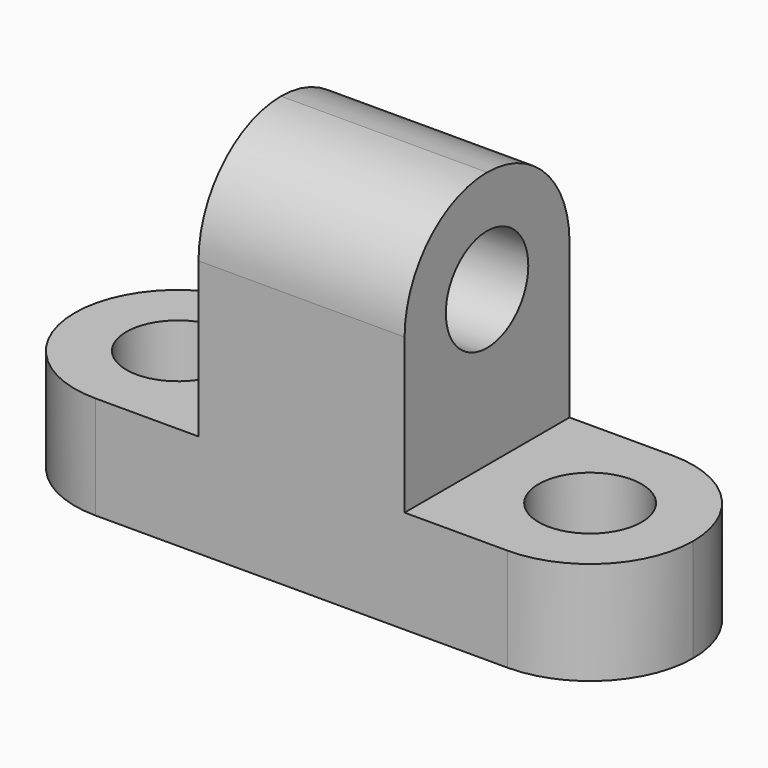
from build123d import *

# Parameters (mm, degrees)
F0_W      = 25.4
F0_H      = 44.45
F1_DEPTH  = 25.4
F2_R      = 12.69999
F3_W      = 25.4
F3_H      = 12.7
F4_DEPTH  = 25.4
F5_R      = 12.69999
F7_W      = 25.4
F7_H      = 12.7
F8_DEPTH  = 25.4
F9_R      = 12.69999
F11_R     = 6.35
F12_DEPTH = 25.4
F6_R      = 6.35
F13_DEPTH = 25.4
F10_R     = 6.35
F14_DEPTH = 25.4


# Not quite as in the source:
# - a fillet or chamfer is up to 0.001 mm smaller than in the source, because OpenCascade refuses the exact size


with BuildPart() as f1:
    # F0 (on Front) → F1 (new body)
    with BuildSketch(Plane.XZ):
        with Locations((12.7, 22.225)):
            Rectangle(F0_W, F0_H)
    extrude(amount=-F1_DEPTH)

    # F2 (radius 12.7 in the source; OpenCascade refuses exactly that, so slightly less here)
    f2_edges = [f1.edges().sort_by_distance(p)[0] for p in [
        (12.7, 0, 44.45),
        (12.7, 25.4, 44.45),
    ]]
    fillet(f2_edges, radius=F2_R)

    # F3 (on face) → F4 (join)
    with BuildSketch(Plane.YZ.offset(25.4)):
        with Locations((12.7, 6.35)):
            Rectangle(F3_W, F3_H)
    extrude(amount=F4_DEPTH)

    # F5 (radius 12.7 in the source; OpenCascade refuses exactly that, so slightly less here)
    f5_edges = [f1.edges().sort_by_distance(p)[0] for p in [
        (50.8, 0, 6.35),
        (50.8, 25.4, 6.35),
    ]]
    fillet(f5_edges, radius=F5_R)

    # F7 (on face) → F8 (join)
    with BuildSketch(Plane(origin=(0, 0, 0), x_dir=(0, -1, 0), z_dir=(-1, 0, 0))):
        with Locations((-12.7, 6.35)):
            Rectangle(F7_W, F7_H)
    extrude(amount=F8_DEPTH)

    # F9 (radius 12.7 in the source; OpenCascade refuses exactly that, so slightly less here)
    f9_edges = [f1.edges().sort_by_distance(p)[0] for p in [
        (-25.4, 25.4, 6.35),
        (-25.4, 0, 6.35),
    ]]
    fillet(f9_edges, radius=F9_R)

    # F11 (on face) → F12 (cut)
    with BuildSketch(Plane.YZ.offset(25.4)):
        with Locations((12.7, 31.75)):
            Circle(F11_R)
    extrude(amount=-F12_DEPTH, mode=Mode.SUBTRACT)

    # F6 (on face) → F13 (cut)
    with BuildSketch(Plane.XY.offset(12.7)):
        with Locations((38.1, 12.7)):
            Circle(F6_R)
    extrude(amount=-F13_DEPTH, mode=Mode.SUBTRACT)

    # F10 (on face) → F14 (cut)
    with BuildSketch(Plane.XY.offset(12.7)):
        with Locations((-12.7, 12.7)):
            Circle(F10_R)
    extrude(amount=-F14_DEPTH, mode=Mode.SUBTRACT)


solid = f1.part
